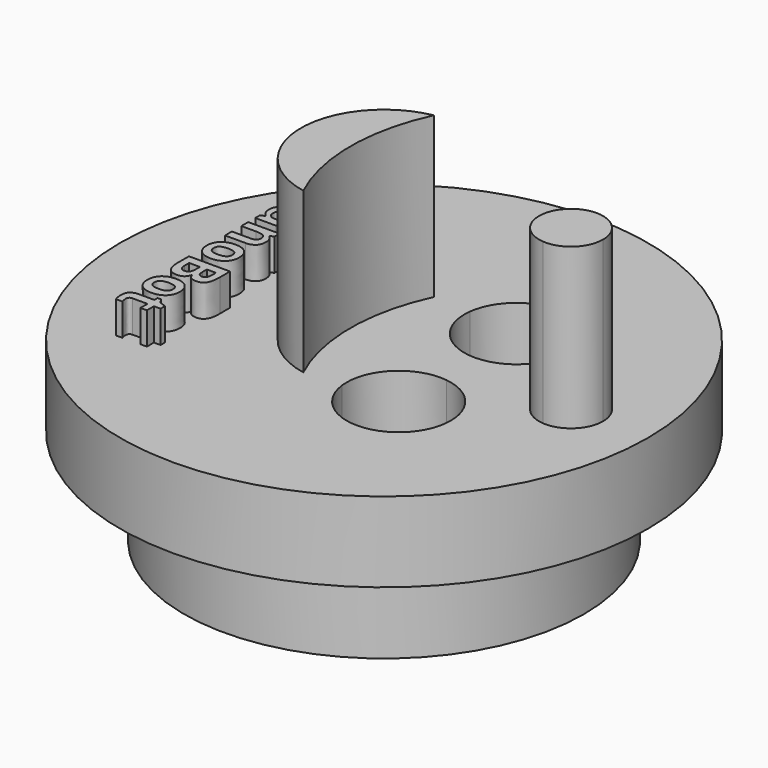
from build123d import *

# Parameters (mm, degrees)
F0_R         = 16.5
F1_DEPTH     = 5
F2_DEPTH     = 10
F3_R         = 12.5
F3_R_2       = 9.5
F4_DEPTH     = 6
F5_DEPTH     = 3.5
F6_TEXT_SIZE = 3.5944959281
F7_DEPTH     = 2


# Not quite as in the source:
# - a feature names something its author has since deleted; it is built from what else it names
# - Text() gives the source's letters only with a copy of the font that has no kerning and outlines rounded to 1/6400 em; it was checked with that copy


with BuildPart() as f1:
    # F0 (on Top) → F1 (new body)
    with BuildSketch(Plane.XY):
        Circle(F0_R)
        with BuildLine():
            ThreePointArc((11.5189136014, -1.9926689249), (-11.69, 0), (11.5189136014, 1.9926689249))
            ThreePointArc((11.5189136014, 1.9926689249), (13.0423733217, 1.4734606878), (13.69, 0))
            ThreePointArc((13.69, 0), (13.0423733217, -1.4734606878), (11.5189136014, -1.9926689249))
        make_face(mode=Mode.SUBTRACT)
        with BuildLine():
            ThreePointArc((11.5189136014, -1.9926689249), (9.69, 0), (11.5189136014, 1.9926689249))
            ThreePointArc((11.5189136014, 1.9926689249), (-11.69, 0), (11.5189136014, -1.9926689249))
        make_face()
        with BuildLine():
            ThreePointArc((-0.9623408959, -5.1), (-5.19, 0), (-0.9623408959, 5.1))
            ThreePointArc((-0.9623408959, 5.1), (0.2102507643, 5.1857395438), (1.3720526533, 5.0053542848))
            ThreePointArc((1.3720526533, 5.0053542848), (4.8011823341, 7.8397229915), (7.8461940777, 4.5961940777))
            ThreePointArc((7.8461940777, 4.5961940777), (7.0346639538, 2.4476213739), (5.0053542848, 1.3720526533))
            ThreePointArc((5.0053542848, 1.3720526533), (5.1436314379, 0.6922106839), (5.19, 0))
            ThreePointArc((5.19, 0), (5.1436314379, -0.6922106839), (5.0053542848, -1.3720526533))
            ThreePointArc((5.0053542848, -1.3720526533), (7.0346639538, -2.4476213739), (7.8461940777, -4.5961940777))
            ThreePointArc((7.8461940777, -4.5961940777), (4.8011823341, -7.8397229915), (1.3720526533, -5.0053542848))
            ThreePointArc((1.3720526533, -5.0053542848), (0.2102507643, -5.1857395438), (-0.9623408959, -5.1))
        make_face(mode=Mode.SUBTRACT)
        with BuildLine():
            ThreePointArc((1.3720526533, 5.0053542848), (0.2102507643, 5.1857395438), (-0.9623408959, 5.1))
            Line((-0.9623408959, 5.1), (-0.9623408959, -5.1))
            ThreePointArc((-0.9623408959, -5.1), (0.2102507643, -5.1857395438), (1.3720526533, -5.0053542848))
            ThreePointArc((1.3720526533, -5.0053542848), (2.2980970389, -2.2980970389), (5.0053542848, -1.3720526533))
            ThreePointArc((5.0053542848, -1.3720526533), (5.1436314379, -0.6922106839), (5.19, 0))
            ThreePointArc((5.19, 0), (5.1436314379, 0.6922106839), (5.0053542848, 1.3720526533))
            ThreePointArc((5.0053542848, 1.3720526533), (2.2980970389, 2.2980970389), (1.3720526533, 5.0053542848))
        make_face()
        with BuildLine():
            ThreePointArc((-0.9623408959, -5.1), (-2.1000207018, 0), (-0.9623408959, 5.1))
            ThreePointArc((-0.9623408959, 5.1), (-5.19, 0), (-0.9623408959, -5.1))
        make_face()
        with BuildLine():
            ThreePointArc((7.8461940777, 4.5961940777), (4.8011823341, 7.8397229915), (1.3720526533, 5.0053542848))
            ThreePointArc((1.3720526533, 5.0053542848), (2.2812284458, 4.6617697045), (3.110401391, 4.1546965217))
            ThreePointArc((3.110401391, 4.1546965217), (4.373123085, 6.1300582608), (6.1461940777, 4.5961940777))
            ThreePointArc((6.1461940777, 4.5961940777), (5.5230648314, 3.3538533008), (4.1546965217, 3.110401391))
            ThreePointArc((4.1546965217, 3.110401391), (4.6617697045, 2.2812284458), (5.0053542848, 1.3720526533))
            ThreePointArc((5.0053542848, 1.3720526533), (7.0346639538, 2.4476213739), (7.8461940777, 4.5961940777))
        make_face()
        with BuildLine():
            ThreePointArc((3.110401391, -4.1546965217), (2.2812284458, -4.6617697045), (1.3720526533, -5.0053542848))
            ThreePointArc((1.3720526533, -5.0053542848), (4.8011823341, -7.8397229915), (7.8461940777, -4.5961940777))
            ThreePointArc((7.8461940777, -4.5961940777), (7.0346639538, -2.4476213739), (5.0053542848, -1.3720526533))
            ThreePointArc((5.0053542848, -1.3720526533), (4.6617697045, -2.2812284458), (4.1546965217, -3.110401391))
            ThreePointArc((4.1546965217, -3.110401391), (5.5230648314, -3.3538533008), (6.1461940777, -4.5961940777))
            ThreePointArc((6.1461940777, -4.5961940777), (4.373123085, -6.1300582608), (3.110401391, -4.1546965217))
        make_face()
        with BuildLine():
            Line((-0.9623408959, -5.1), (-0.9623408959, 5.1))
            ThreePointArc((-0.9623408959, 5.1), (-2.1000207018, 0), (-0.9623408959, -5.1))
        make_face()
        with BuildLine():
            ThreePointArc((3.110401391, 4.1546965217), (2.2812284458, 4.6617697045), (1.3720526533, 5.0053542848))
            ThreePointArc((1.3720526533, 5.0053542848), (2.2980970389, 2.2980970389), (5.0053542848, 1.3720526533))
            ThreePointArc((5.0053542848, 1.3720526533), (4.6617697045, 2.2812284458), (4.1546965217, 3.110401391))
            ThreePointArc((4.1546965217, 3.110401391), (3.5001785669, 3.5001785669), (3.110401391, 4.1546965217))
        make_face()
        with BuildLine():
            ThreePointArc((5.0053542848, -1.3720526533), (2.2980970389, -2.2980970389), (1.3720526533, -5.0053542848))
            ThreePointArc((1.3720526533, -5.0053542848), (2.2812284458, -4.6617697045), (3.110401391, -4.1546965217))
            ThreePointArc((3.110401391, -4.1546965217), (3.5001785669, -3.5001785669), (4.1546965217, -3.110401391))
            ThreePointArc((4.1546965217, -3.110401391), (4.6617697045, -2.2812284458), (5.0053542848, -1.3720526533))
        make_face()
        with BuildLine():
            ThreePointArc((11.5189136014, 1.9926689249), (11.647149866, 1), (11.69, 0))
            ThreePointArc((11.69, 0), (11.647149866, -1), (11.5189136014, -1.9926689249))
            ThreePointArc((11.5189136014, -1.9926689249), (13.0423733217, -1.4734606878), (13.69, 0))
            ThreePointArc((13.69, 0), (13.0423733217, 1.4734606878), (11.5189136014, 1.9926689249))
        make_face()
        with BuildLine():
            ThreePointArc((11.5189136014, -1.9926689249), (11.647149866, -1), (11.69, 0))
            ThreePointArc((11.69, 0), (11.647149866, 1), (11.5189136014, 1.9926689249))
            ThreePointArc((11.5189136014, 1.9926689249), (9.69, 0), (11.5189136014, -1.9926689249))
        make_face()
    extrude(amount=-F1_DEPTH)

    # F0 (on Top) → F2 (join)
    with BuildSketch(Plane.XY):
        with BuildLine():
            ThreePointArc((11.5189136014, 1.9926689249), (11.647149866, 1), (11.69, 0))
            ThreePointArc((11.69, 0), (11.647149866, -1), (11.5189136014, -1.9926689249))
            ThreePointArc((11.5189136014, -1.9926689249), (13.0423733217, -1.4734606878), (13.69, 0))
            ThreePointArc((13.69, 0), (13.0423733217, 1.4734606878), (11.5189136014, 1.9926689249))
        make_face()
        with BuildLine():
            ThreePointArc((11.5189136014, -1.9926689249), (11.647149866, -1), (11.69, 0))
            ThreePointArc((11.69, 0), (11.647149866, 1), (11.5189136014, 1.9926689249))
            ThreePointArc((11.5189136014, 1.9926689249), (9.69, 0), (11.5189136014, -1.9926689249))
        make_face()
        with BuildLine():
            ThreePointArc((-0.9623408959, -5.1), (-2.1000207018, 0), (-0.9623408959, 5.1))
            ThreePointArc((-0.9623408959, 5.1), (-5.19, 0), (-0.9623408959, -5.1))
        make_face()
    extrude(amount=F2_DEPTH)

    # F3 (on face) → F4 (join)
    with BuildSketch(Plane(origin=(0, 0, -5), x_dir=(1, 0, 0), z_dir=(0, 0, -1))):
        Circle(F3_R)
        Circle(F3_R_2, mode=Mode.SUBTRACT)
    extrude(amount=F4_DEPTH)

    # F0 (on Top) → F5 (cut)
    with BuildSketch(Plane.XY):
        with BuildLine():
            ThreePointArc((3.110401391, -4.1546965217), (2.2812284458, -4.6617697045), (1.3720526533, -5.0053542848))
            ThreePointArc((1.3720526533, -5.0053542848), (4.8011823341, -7.8397229915), (7.8461940777, -4.5961940777))
            ThreePointArc((7.8461940777, -4.5961940777), (7.0346639538, -2.4476213739), (5.0053542848, -1.3720526533))
            ThreePointArc((5.0053542848, -1.3720526533), (4.6617697045, -2.2812284458), (4.1546965217, -3.110401391))
            ThreePointArc((4.1546965217, -3.110401391), (5.5230648314, -3.3538533008), (6.1461940777, -4.5961940777))
            ThreePointArc((6.1461940777, -4.5961940777), (4.373123085, -6.1300582608), (3.110401391, -4.1546965217))
        make_face()
        with BuildLine():
            ThreePointArc((5.0053542848, -1.3720526533), (2.2980970389, -2.2980970389), (1.3720526533, -5.0053542848))
            ThreePointArc((1.3720526533, -5.0053542848), (2.2812284458, -4.6617697045), (3.110401391, -4.1546965217))
            ThreePointArc((3.110401391, -4.1546965217), (3.5001785669, -3.5001785669), (4.1546965217, -3.110401391))
            ThreePointArc((4.1546965217, -3.110401391), (4.6617697045, -2.2812284458), (5.0053542848, -1.3720526533))
        make_face()
        with BuildLine():
            ThreePointArc((4.1546965217, -3.110401391), (3.5001785669, -3.5001785669), (3.110401391, -4.1546965217))
            ThreePointArc((3.110401391, -4.1546965217), (3.6698841944, -3.6698841944), (4.1546965217, -3.110401391))
        make_face()
        with BuildLine():
            ThreePointArc((7.8461940777, 4.5961940777), (4.8011823341, 7.8397229915), (1.3720526533, 5.0053542848))
            ThreePointArc((1.3720526533, 5.0053542848), (2.2812284458, 4.6617697045), (3.110401391, 4.1546965217))
            ThreePointArc((3.110401391, 4.1546965217), (4.373123085, 6.1300582608), (6.1461940777, 4.5961940777))
            ThreePointArc((6.1461940777, 4.5961940777), (5.5230648314, 3.3538533008), (4.1546965217, 3.110401391))
            ThreePointArc((4.1546965217, 3.110401391), (4.6617697045, 2.2812284458), (5.0053542848, 1.3720526533))
            ThreePointArc((5.0053542848, 1.3720526533), (7.0346639538, 2.4476213739), (7.8461940777, 4.5961940777))
        make_face()
        with BuildLine():
            ThreePointArc((3.110401391, 4.1546965217), (2.2812284458, 4.6617697045), (1.3720526533, 5.0053542848))
            ThreePointArc((1.3720526533, 5.0053542848), (2.2980970389, 2.2980970389), (5.0053542848, 1.3720526533))
            ThreePointArc((5.0053542848, 1.3720526533), (4.6617697045, 2.2812284458), (4.1546965217, 3.110401391))
            ThreePointArc((4.1546965217, 3.110401391), (3.5001785669, 3.5001785669), (3.110401391, 4.1546965217))
        make_face()
        with BuildLine():
            ThreePointArc((4.1546965217, 3.110401391), (3.6698841944, 3.6698841944), (3.110401391, 4.1546965217))
            ThreePointArc((3.110401391, 4.1546965217), (3.5001785669, 3.5001785669), (4.1546965217, 3.110401391))
        make_face()
    extrude(amount=-F5_DEPTH, mode=Mode.SUBTRACT)

    # F6 (on face) → F7 (join)
    with BuildSketch(Plane.XY):
        with Locations(Location((-10.5880370682, 8), (0, 0, -90))):
            Text('NanoBot', F6_TEXT_SIZE, font='Open Sans', font_style=FontStyle.BOLD, text_align=(TextAlign.LEFT, TextAlign.BOTTOM))
    extrude(amount=F7_DEPTH)


solid = f1.part
